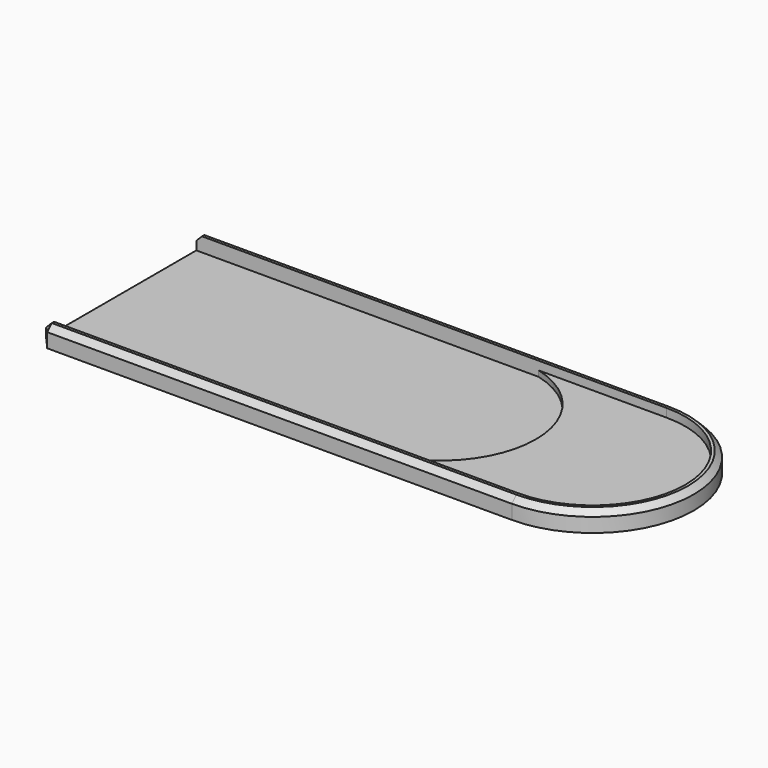
from build123d import *

# Parameters (mm, degrees)
F0_W     = 145.3
F0_H     = 65
F1_DEPTH = 2
F0_W_2   = 20
F3_DEPTH = 4
F4_DEPTH = 2
F0_H_2   = 3
F5_DEPTH = 7
F6_DEPTH = 7
F7_SIZE  = 1.99999


# Not quite as in the source:
# - a fillet or chamfer is up to 0.001 mm smaller than in the source, because OpenCascade refuses the exact size


with BuildPart() as f1:
    # F0 (on Top) → F1 (new body)
    with BuildSketch(Plane.XY):
        Rectangle(F0_W, F0_H)
    extrude(amount=F1_DEPTH)

    # F0 (on Top) → F3 (join)
    with BuildSketch(Plane.XY):
        with Locations((82.65, 0)):
            Rectangle(F0_W_2, F0_H)
        with BuildLine():
            ThreePointArc((92.65, -32.5), (125.15, 0), (92.65, 32.5))
            Line((92.65, 32.5), (92.65, -32.5))
        make_face()
    extrude(amount=F3_DEPTH)

    # F2 (on face) → F4 (join)
    with BuildSketch(Plane.XY.offset(2)):
        with BuildLine():
            ThreePointArc((47.65, 32.5), (65.6769816336, 20.5015243336), (72.65, 0))
            Line((72.65, 0), (72.65, 32.5))
            Line((72.65, 32.5), (47.65, 32.5))
        make_face()
        with BuildLine():
            ThreePointArc((72.65, 0), (65.6769816336, -20.5015243336), (47.65, -32.5))
            Line((47.65, -32.5), (72.65, -32.5))
            Line((72.65, -32.5), (72.65, 0))
        make_face()
    extrude(amount=F4_DEPTH)

    # F0 (on Top) → F5 (join)
    with BuildSketch(Plane.XY):
        with BuildLine():
            Line((92.65, 35.5), (92.65, 32.5))
            ThreePointArc((92.65, 32.5), (125.15, 0), (92.65, -32.5))
            Line((92.65, -32.5), (92.65, -35.5))
            ThreePointArc((92.65, -35.5), (128.15, 0), (92.65, 35.5))
        make_face()
        with Locations((82.65, -34)):
            Rectangle(F0_W_2, F0_H_2)
        with Locations((82.65, 34)):
            Rectangle(F0_W_2, F0_H_2)
    extrude(amount=F5_DEPTH)

    # F0 (on Top) → F6 (join)
    with BuildSketch(Plane.XY):
        with Locations((0, -34)):
            Rectangle(F0_W, F0_H_2)
        with Locations((0, 34)):
            Rectangle(F0_W, F0_H_2)
    extrude(amount=F6_DEPTH)

    # F7 (size 2 in the source; OpenCascade refuses exactly that, so slightly less here)
    f7_edges = [f1.edges().sort_by_distance(p)[0] for p in [
        (-72.65, 35.5, 3.5),
        (-72.65, -35.5, 3.5),
        (-72.65, -34, 7),
        (-72.65, 34, 7),
        (-72.65, 0, 0),
        (10, 35.5, 7),
    ]]
    chamfer(f7_edges, length=F7_SIZE)


solid = f1.part
